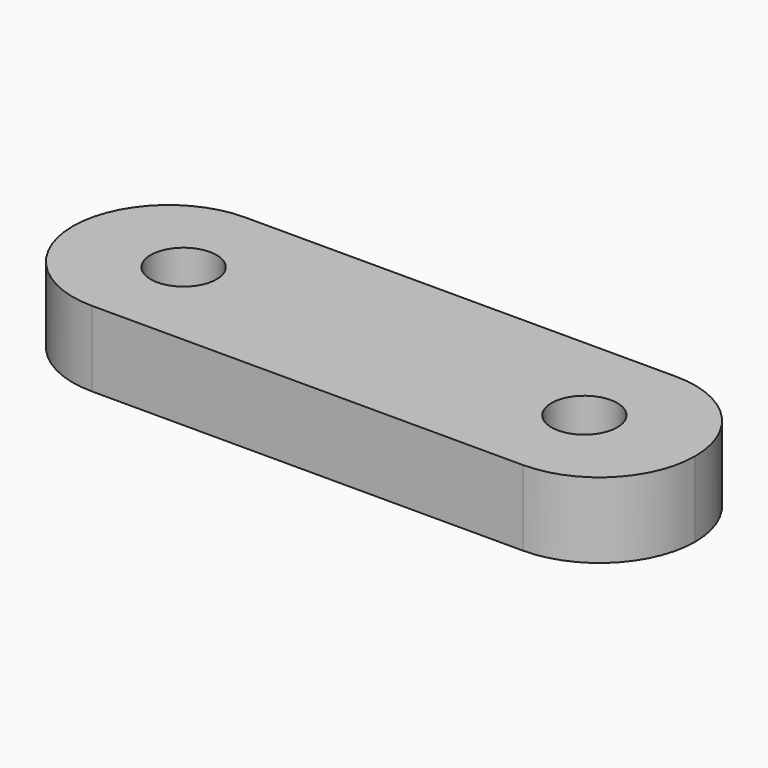
from build123d import *

# Parameters (mm, degrees)
F0_W     = 41.275
F0_H     = 12.7
F1_DEPTH = 5
F2_R     = 2.1845
F2_R_2   = 2.1844
F3_DEPTH = 25
F4_R     = 6.34999


# Not quite as in the source:
# - a fillet or chamfer is up to 0.001 mm smaller than in the source, because OpenCascade refuses the exact size


with BuildPart() as f1:
    # F0 (on Top) → F1 (new body)
    with BuildSketch(Plane.XY):
        with Locations((0.7436354645, -0.3860430318)):
            Rectangle(F0_W, F0_H)
    extrude(amount=F1_DEPTH)

    # F2 (on face) → F3 (cut)
    with BuildSketch(Plane(origin=(0, 0, 0), x_dir=(1, 0, 0), z_dir=(0, 0, -1))):
        with Locations((-12.5438645355, 0.3860430318)):
            Circle(F2_R)
        with Locations((14.0311354645, 0.3860430318)):
            Circle(F2_R_2)
    extrude(amount=-F3_DEPTH, mode=Mode.SUBTRACT)

    # F4 (radius 6.35 in the source; OpenCascade refuses exactly that, so slightly less here)
    f4_edges = [f1.edges().sort_by_distance(p)[0] for p in [
        (21.381135, -6.736043, 2.5),
        (21.381135, 5.963957, 2.5),
        (-19.893865, -6.736043, 2.5),
        (-19.893865, 5.963957, 2.5),
    ]]
    fillet(f4_edges, radius=F4_R)


solid = f1.part
